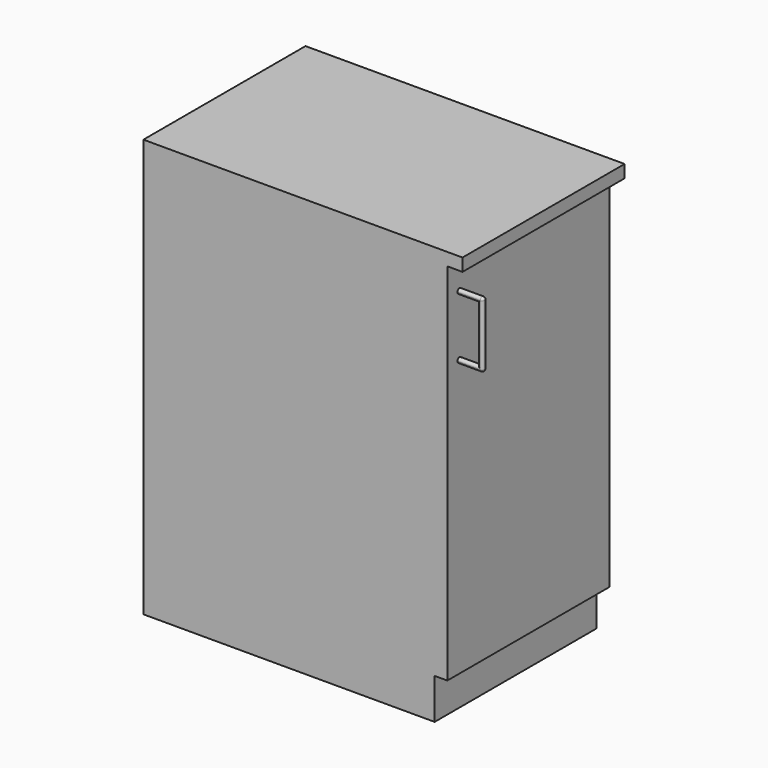
from build123d import *

# Parameters (mm, degrees)
F0_W        = 600
F0_H        = 400
F1_DEPTH    = 800
F2_W        = 400
F2_H        = 80
F3_DEPTH    = 25
F5_DEPTH    = 50
F6_T1_DEPTH = 120
F6_T4_ANGLE = 180
F6_T6_ANGLE = 180
F7_W        = 40
F7_H        = 110
F8_DEPTH    = 25
F9_R        = 4.99999
F10_W       = 630
F10_H       = 400
F11_DEPTH   = 25


# Not quite as in the source:
# - a fillet or chamfer that OpenCascade refuses, or shapes differently, is made with other operations: its cross-section is extruded or revolved along the edge and cut away or added
# - a fillet or chamfer is up to 0.001 mm smaller than in the source, because OpenCascade refuses the exact size


with BuildPart() as f1:
    # F0 (on Top) → F1 (new body)
    with BuildSketch(Plane.XY):
        Rectangle(F0_W, F0_H)
    extrude(amount=F1_DEPTH)

    # F2 (on face) → F3 (cut)
    with BuildSketch(Plane.YZ.offset(300)):
        with Locations((0, 40)):
            Rectangle(F2_W, F2_H)
    extrude(amount=-F3_DEPTH, mode=Mode.SUBTRACT)

    # F4 (on face) → F5 (join)
    with BuildSketch(Plane.YZ.offset(300)):
        with BuildLine():
            ThreePointArc((-170, 750), (-173.5355339059, 748.5355339059), (-175, 745))
            Line((-175, 745), (-175, 625))
            ThreePointArc((-175, 625), (-173.5355339059, 621.4644660941), (-170, 620))
            ThreePointArc((-170, 620), (-166.4644660941, 621.4644660941), (-165, 625))
            Line((-165, 625), (-165, 745))
            ThreePointArc((-165, 745), (-166.4644660941, 748.5355339059), (-170, 750))
        make_face()
    extrude(amount=F5_DEPTH)

    # F6: fillet of radius 5 on 4 edges, made by hand

    # F6_s2 → F6_t1 (cut)
    with BuildSketch(Plane.XY.offset(625)):
        with BuildLine():
            ThreePointArc((345, -175), (348.5355339059, -173.5355339059), (350, -170))
            Line((350, -170), (350, -175))
            Line((350, -175), (345, -175))
        make_face()
        with BuildLine():
            ThreePointArc((345, -165), (348.5355339059, -166.4644660941), (350, -170))
            Line((350, -170), (350, -165))
            Line((350, -165), (345, -165))
        make_face()
    extrude(amount=F6_T1_DEPTH, mode=Mode.SUBTRACT)

    # F6_s3 → F6_t4 (revolve, cut)
    with BuildSketch(Plane.XY.offset(745)):
        with BuildLine():
            ThreePointArc((345, -175), (348.5355339059, -173.5355339059), (350, -170))
            Line((350, -170), (350, -175))
            Line((350, -175), (345, -175))
        make_face()
    revolve(axis=Axis((350, -170, 745), (-1, 0, 0)), revolution_arc=F6_T4_ANGLE, mode=Mode.SUBTRACT)

    # F6_s5 → F6_t6 (revolve, cut)
    with BuildSketch(Plane.XY.offset(625)):
        with BuildLine():
            ThreePointArc((345, -165), (348.5355339059, -166.4644660941), (350, -170))
            Line((350, -170), (350, -165))
            Line((350, -165), (345, -165))
        make_face()
    revolve(axis=Axis((350, -170, 625), (-1, 0, 0)), revolution_arc=F6_T6_ANGLE, mode=Mode.SUBTRACT)

    # F7 (on face) → F8 (cut)
    with BuildSketch(Plane(origin=(0, -165, 0), x_dir=(-1, 0, 0), z_dir=(0, 1, 0))):
        with Locations((-320, 685)):
            Rectangle(F7_W, F7_H)
    extrude(amount=-F8_DEPTH, mode=Mode.SUBTRACT)

    # F9 (radius 5 in the source; OpenCascade refuses exactly that, so slightly less here)
    f9_edges = [f1.edges().sort_by_distance(p)[0] for p in [
        (320, -165, 740),
        (340, -165, 685),
        (320, -165, 630),
        (320, -175, 740),
        (340, -175, 685),
        (320, -175, 630),
    ]]
    fillet(f9_edges, radius=F9_R)

    # F10 (on face) → F11 (join)
    with BuildSketch(Plane.XY.offset(800)):
        with Locations((15, 0)):
            Rectangle(F10_W, F10_H)
    extrude(amount=F11_DEPTH)


solid = f1.part
